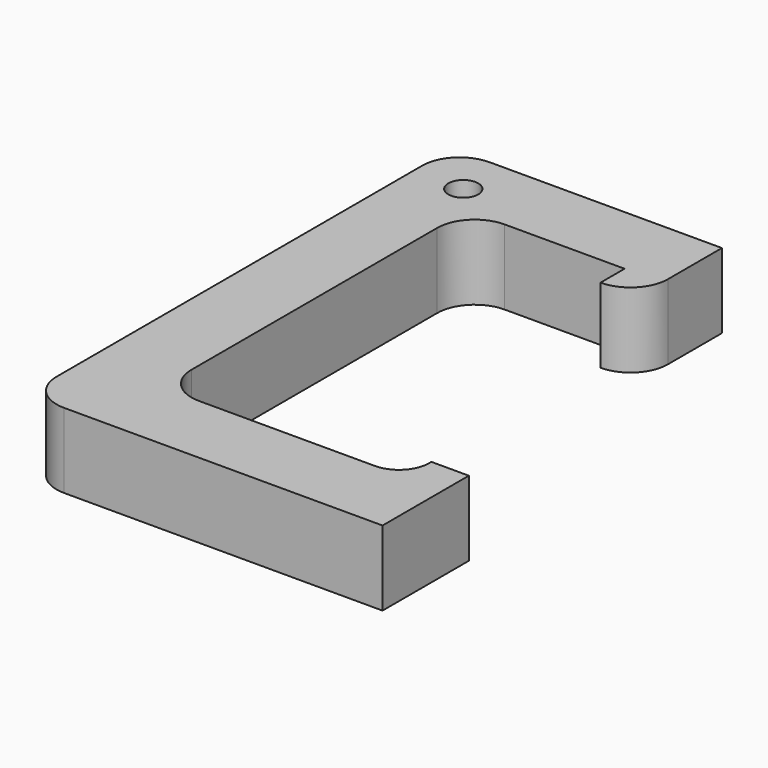
from build123d import *

# Parameters (mm, degrees)
F1_DEPTH = 10
F2_R     = 5
F3_R     = 4.99999
F5_R     = 4
F6_R     = 2
F7_DEPTH = 10


# Not quite as in the source:
# - two fillets or chamfers of one size are made in one step
# - a fillet or chamfer is up to 0.001 mm smaller than in the source, because OpenCascade refuses the exact size


with BuildPart() as f1:
    # F0 (on Top) → F1 (new body)
    with BuildSketch(Plane.XY):
        Polygon((0, 70.9848281697), (0, 0), (36, 0), (47.5, 0), (47.5, 14.3951736391), (42.5, 14.3951736391), (42.5, 10), (36, 10), (10, 10), (10, 61), (26.8777515739, 61), (31, 61), (31, 56.9848281697), (36, 56.9848281697), (36, 70.9848281697), align=None)
    extrude(amount=F1_DEPTH)

    # F2
    f2_edges = [f1.edges().sort_by_distance(p)[0] for p in [
        (0, 0, 5),
        (0, 70.984828, 5),
    ]]
    fillet(f2_edges, radius=F2_R)

    # F3 (radius 5 in the source; OpenCascade refuses exactly that, so slightly less here)
    f3_edges = [f1.edges().sort_by_distance(p)[0] for p in [
        (10, 10, 5),
        (36, 56.984828, 5),
        (10, 61, 5),
    ]]
    fillet(f3_edges, radius=F3_R)

    # F5
    f5_edges = [f1.edges().sort_by_distance(p)[0] for p in [
        (42.5, 10, 5),
    ]]
    fillet(f5_edges, radius=F5_R)

    # F6 (on face) → F7 (cut, through all)
    with BuildSketch(Plane.XY.offset(10)):
        with Locations((6.6156452522, 64.5774751902)):
            Circle(F6_R)
    extrude(amount=-F7_DEPTH, mode=Mode.SUBTRACT)


solid = f1.part
